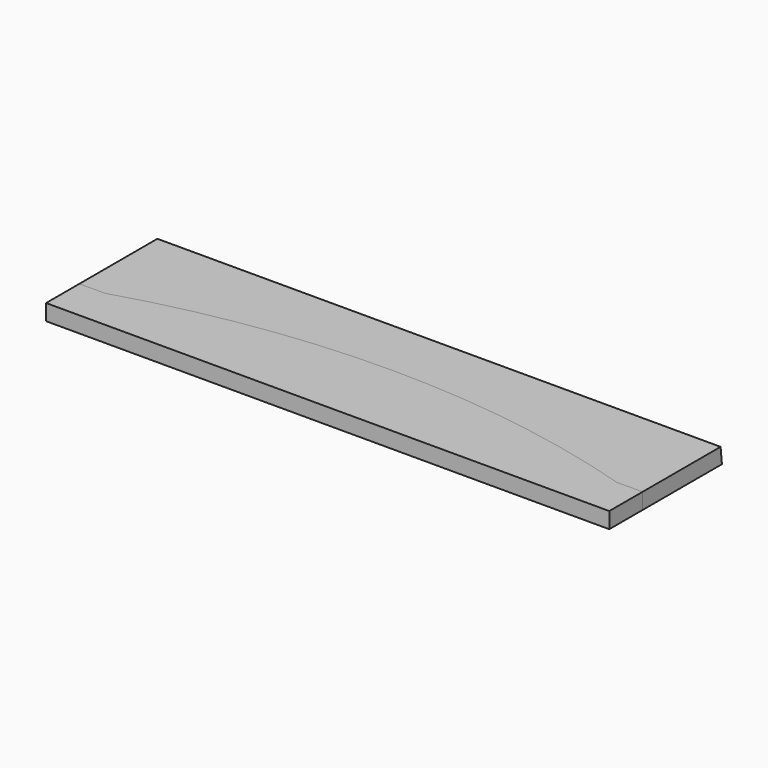
from build123d import *

# Parameters (mm, degrees)
F1_DEPTH = 15.875
F2_DEPTH = 15.875
F3_SIZE2 = 1.66852
F3_SIZE  = 15.87499


# Not quite as in the source:
# - a fillet or chamfer is up to 0.001 mm smaller than in the source, because OpenCascade refuses the exact size


with BuildPart() as f1:
    # F0 (on Top) → F1 (new body)
    with BuildSketch(Plane.XY):
        with BuildLine():
            Line((558.8, 0), (0, 0))
            Line((0, 0), (0, -98.425))
            Line((0, -98.425), (25.4, -98.425))
            ThreePointArc((25.4, -98.425), (279.4, -60.325), (533.4, -98.425))
            Line((533.4, -98.425), (558.8, -98.425))
            Line((558.8, -98.425), (558.8, 0))
        make_face()
    extrude(amount=F1_DEPTH)

    # F3 (size 15.875 and 1.6685297348 in the source; OpenCascade refuses exactly that, so slightly less here)
    f3_edges = [f1.edges().sort_by_distance(p)[0] for p in [
        (279.4, 0, 15.875),
    ]]
    f3_side = f1.faces().sort_by_distance((279.4, 0, 7.9375))[0]
    chamfer(f3_edges, length=F3_SIZE, length2=F3_SIZE2, reference=f3_side)


with BuildPart() as f2:
    # F0 (on Top) → F2 (new body)
    with BuildSketch(Plane.XY):
        with BuildLine():
            Line((25.4, -98.425), (0, -98.425))
            Line((0, -98.425), (0, -139.7))
            Line((0, -139.7), (558.8, -139.7))
            Line((558.8, -139.7), (558.8, -98.425))
            Line((558.8, -98.425), (533.4, -98.425))
            ThreePointArc((533.4, -98.425), (279.4, -60.325), (25.4, -98.425))
        make_face()
    extrude(amount=F2_DEPTH)


solid = Compound([f1.part, f2.part])
